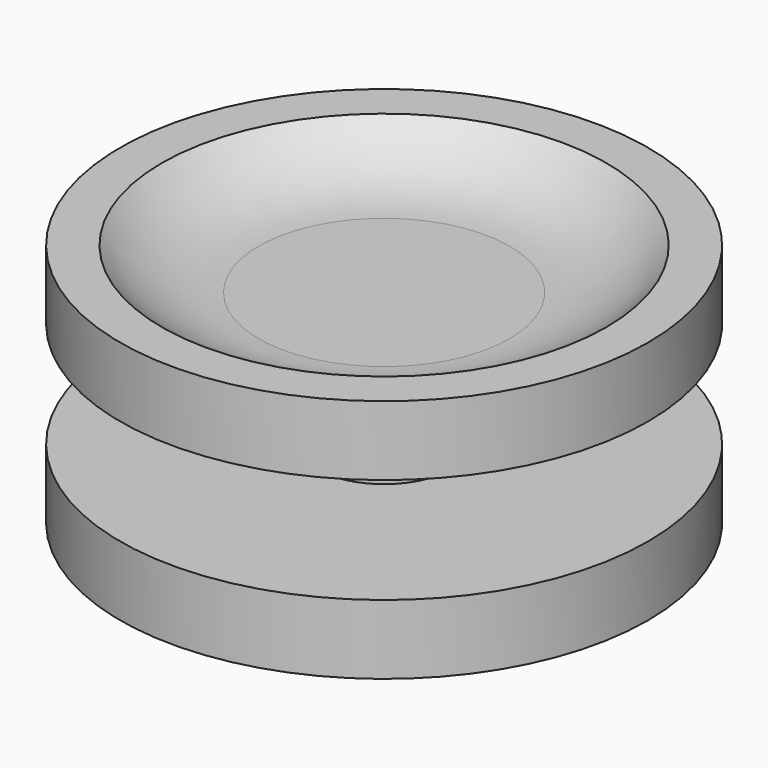
from build123d import *

# Parameters (mm, degrees)
F0_R      = 3.1115
F0_R_2    = 2.0743333333
F1_DEPTH  = 4.826
F2_R      = 12.065
F3_DEPTH  = 3.175
F4_R      = 10.16
F5_DEPTH  = 1.905
F6_R      = 2.0489333333
F7_DEPTH  = 4.826
F8_R      = 12.065
F9_DEPTH  = 3.175
F10_R     = 10.16
F11_DEPTH = 1.905


# Not quite as in the source:
# - a fillet or chamfer that OpenCascade refuses, or shapes differently, is made with other operations: its cross-section is extruded or revolved along the edge and cut away or added


with BuildPart() as f1:
    # F0 (on Top) → F1 (new body)
    with BuildSketch(Plane.XY):
        Circle(F0_R)
        Circle(F0_R_2, mode=Mode.SUBTRACT)
    extrude(amount=F1_DEPTH)

    # F2 (on face) → F3 (join)
    with BuildSketch(Plane.XY.offset(4.826)):
        Circle(F2_R)
    extrude(amount=F3_DEPTH)

    # F4 (on face) → F5 (cut)
    with BuildSketch(Plane.XY.offset(8.001)):
        Circle(F4_R)
    extrude(amount=-F5_DEPTH, mode=Mode.SUBTRACT)

    # F12: fillet of radius 6.096 on 1 edges, made by hand

    # F12_s1 → F12_t2 (revolve)
    with BuildSketch(Plane.XZ):
        with BuildLine():
            ThreePointArc((10.16, 8.001), (8.1428356123, 6.592466448), (5.7331800353, 6.096))
            Line((5.7331800353, 6.096), (10.16, 6.096))
            Line((10.16, 6.096), (10.16, 8.001))
        make_face()
    revolve(axis=Axis((0, 0, 6.096), (0, 0, 1)))


with BuildPart() as f7:
    # F6 (on face) → F7 (new body)
    with BuildSketch(Plane(origin=(0, 0, 0), x_dir=(1, 0, 0), z_dir=(0, 0, -1))):
        Circle(F6_R)
    extrude(amount=-F7_DEPTH)

    # F8 (on face) → F9 (join)
    with BuildSketch(Plane(origin=(0, 0, 0), x_dir=(1, 0, 0), z_dir=(0, 0, -1))):
        Circle(F8_R)
    extrude(amount=F9_DEPTH)

    # F10 (on face) → F11 (cut)
    with BuildSketch(Plane(origin=(0, 0, -3.175), x_dir=(1, 0, 0), z_dir=(0, 0, -1))):
        Circle(F10_R)
    extrude(amount=-F11_DEPTH, mode=Mode.SUBTRACT)

    # F12#2: fillet of radius 6.096 on 1 edges, made by hand

    # F12_2_s1 → F12_2_t2 (revolve)
    with BuildSketch(Plane.XZ):
        with BuildLine():
            ThreePointArc((10.16, -3.175), (8.1428356123, -1.766466448), (5.7331800353, -1.27))
            Line((5.7331800353, -1.27), (10.16, -1.27))
            Line((10.16, -1.27), (10.16, -3.175))
        make_face()
    revolve(axis=Axis((0, 0, -1.27), (0, 0, -1)))


solid = Compound([f1.part, f7.part])
